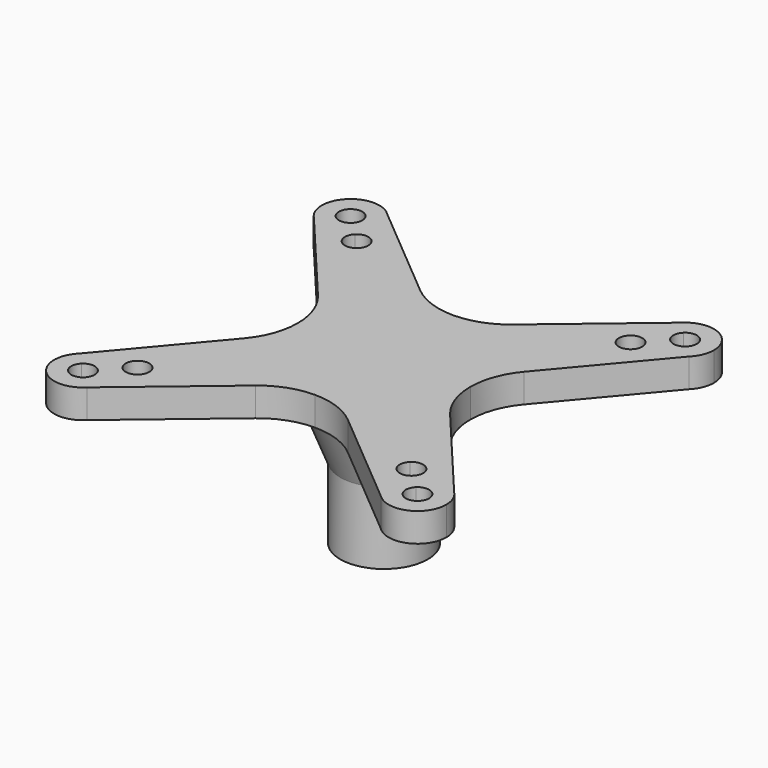
from build123d import *

# Parameters (mm, degrees)
F1_DEPTH = 2.032
F2_DEPTH = 4.572
F4_DEPTH = 5.08


# Not quite as in the source:
# - a fillet or chamfer that OpenCascade refuses, or shapes differently, is made with other operations: its cross-section is extruded or revolved along the edge and cut away or added


with BuildPart() as f1:
    # F0 (on Top) → F1 (new body)
    with BuildSketch(Plane.XY):
        with BuildLine():
            Line((-11.2145823858, 12.3820156815), (-10.3614580543, 13.235140013))
            ThreePointArc((-10.3614580543, 13.235140013), (-13.235140013, 13.235140013), (-13.235140013, 10.3614580543))
            Line((-13.235140013, 10.3614580543), (-12.3820156815, 11.2145823858))
            ThreePointArc((-12.3820156815, 11.2145823858), (-12.3820156815, 12.3820156815), (-11.2145823858, 12.3820156815))
        make_face()
        with BuildLine():
            ThreePointArc((13.8302990336, 11.7982990336), (12.5759117682, 13.6756222437), (10.3614580543, 13.235140013))
            Line((10.3614580543, 13.235140013), (11.2145823858, 12.3820156815))
            ThreePointArc((11.2145823858, 12.3820156815), (12.1142042071, 12.5609615877), (12.6237990336, 11.7982990336))
            ThreePointArc((12.6237990336, 11.7982990336), (12.5609615877, 11.4823938602), (12.3820156815, 11.2145823858))
            Line((12.3820156815, 11.2145823858), (13.235140013, 10.3614580543))
            ThreePointArc((13.235140013, 10.3614580543), (13.6756222437, 11.0206862991), (13.8302990336, 11.7982990336))
        make_face()
        with BuildLine():
            ThreePointArc((13.8302990336, -11.7982990336), (13.6756222437, -11.0206862991), (13.235140013, -10.3614580543))
            Line((13.235140013, -10.3614580543), (12.3820156815, -11.2145823858))
            ThreePointArc((12.3820156815, -11.2145823858), (12.5609615877, -11.4823938602), (12.6237990336, -11.7982990336))
            ThreePointArc((12.6237990336, -11.7982990336), (12.1142042071, -12.5609615877), (11.2145823858, -12.3820156815))
            Line((11.2145823858, -12.3820156815), (10.3614580543, -13.235140013))
            ThreePointArc((10.3614580543, -13.235140013), (12.5759117682, -13.6756222437), (13.8302990336, -11.7982990336))
        make_face()
        with BuildLine():
            Line((-12.3820156815, -11.2145823858), (-13.235140013, -10.3614580543))
            ThreePointArc((-13.235140013, -10.3614580543), (-13.235140013, -13.235140013), (-10.3614580543, -13.235140013))
            Line((-10.3614580543, -13.235140013), (-11.2145823858, -12.3820156815))
            ThreePointArc((-11.2145823858, -12.3820156815), (-12.3820156815, -12.3820156815), (-12.3820156815, -11.2145823858))
        make_face()
        with BuildLine():
            Line((-12.3820156815, 11.2145823858), (-13.235140013, 10.3614580543))
            ThreePointArc((-13.235140013, 10.3614580543), (-11.7982990336, 9.7662990336), (-10.3614580543, 10.3614580543))
            Line((-10.3614580543, 10.3614580543), (-11.2145823858, 11.2145823858))
            ThreePointArc((-11.2145823858, 11.2145823858), (-11.7982990336, 10.9727990336), (-12.3820156815, 11.2145823858))
        make_face()
        with BuildLine():
            ThreePointArc((-9.7662990336, 11.7982990336), (-9.9209758236, 12.5759117682), (-10.3614580543, 13.235140013))
            Line((-10.3614580543, 13.235140013), (-11.2145823858, 12.3820156815))
            ThreePointArc((-11.2145823858, 12.3820156815), (-11.0356364796, 12.1142042071), (-10.9727990336, 11.7982990336))
            ThreePointArc((-10.9727990336, 11.7982990336), (-11.0356364796, 11.4823938602), (-11.2145823858, 11.2145823858))
            Line((-11.2145823858, 11.2145823858), (-10.3614580543, 10.3614580543))
            ThreePointArc((-10.3614580543, 10.3614580543), (-9.9209758236, 11.0206862991), (-9.7662990336, 11.7982990336))
        make_face()
        with BuildLine():
            Line((11.2145823858, 12.3820156815), (10.3614580543, 13.235140013))
            ThreePointArc((10.3614580543, 13.235140013), (9.7662990336, 11.7982990336), (10.3614580543, 10.3614580543))
            Line((10.3614580543, 10.3614580543), (11.2145823858, 11.2145823858))
            ThreePointArc((11.2145823858, 11.2145823858), (10.9727990336, 11.7982990336), (11.2145823858, 12.3820156815))
        make_face()
        with BuildLine():
            Line((11.2145823858, 11.2145823858), (10.3614580543, 10.3614580543))
            ThreePointArc((10.3614580543, 10.3614580543), (11.7982990336, 9.7662990336), (13.235140013, 10.3614580543))
            Line((13.235140013, 10.3614580543), (12.3820156815, 11.2145823858))
            ThreePointArc((12.3820156815, 11.2145823858), (11.7982990336, 10.9727990336), (11.2145823858, 11.2145823858))
        make_face()
        with BuildLine():
            Line((12.3820156815, -11.2145823858), (13.235140013, -10.3614580543))
            ThreePointArc((13.235140013, -10.3614580543), (11.7982990336, -9.7662990336), (10.3614580543, -10.3614580543))
            Line((10.3614580543, -10.3614580543), (11.2145823858, -11.2145823858))
            ThreePointArc((11.2145823858, -11.2145823858), (11.7982990336, -10.9727990336), (12.3820156815, -11.2145823858))
        make_face()
        with BuildLine():
            ThreePointArc((10.3614580543, -10.3614580543), (9.7662990336, -11.7982990336), (10.3614580543, -13.235140013))
            Line((10.3614580543, -13.235140013), (11.2145823858, -12.3820156815))
            ThreePointArc((11.2145823858, -12.3820156815), (10.9727990336, -11.7982990336), (11.2145823858, -11.2145823858))
            Line((11.2145823858, -11.2145823858), (10.3614580543, -10.3614580543))
        make_face()
        with BuildLine():
            Line((-11.2145823858, -12.3820156815), (-10.3614580543, -13.235140013))
            ThreePointArc((-10.3614580543, -13.235140013), (-9.9209758236, -12.5759117682), (-9.7662990336, -11.7982990336))
            ThreePointArc((-9.7662990336, -11.7982990336), (-9.9209758236, -11.0206862991), (-10.3614580543, -10.3614580543))
            Line((-10.3614580543, -10.3614580543), (-11.2145823858, -11.2145823858))
            ThreePointArc((-11.2145823858, -11.2145823858), (-11.0356364796, -11.4823938602), (-10.9727990336, -11.7982990336))
            ThreePointArc((-10.9727990336, -11.7982990336), (-11.0356364796, -12.1142042071), (-11.2145823858, -12.3820156815))
        make_face()
        with BuildLine():
            ThreePointArc((-10.3614580543, -10.3614580543), (-11.7982990336, -9.7662990336), (-13.235140013, -10.3614580543))
            Line((-13.235140013, -10.3614580543), (-12.3820156815, -11.2145823858))
            ThreePointArc((-12.3820156815, -11.2145823858), (-11.7982990336, -10.9727990336), (-11.2145823858, -11.2145823858))
            Line((-11.2145823858, -11.2145823858), (-10.3614580543, -10.3614580543))
        make_face()
        with BuildLine():
            Line((-5.2672343618, 5.2672343618), (-3.2639, 7.2705687236))
            Line((-3.2639, 7.2705687236), (-10.3614580543, 13.235140013))
            ThreePointArc((-10.3614580543, 13.235140013), (-9.9209758236, 12.5759117682), (-9.7662990336, 11.7982990336))
            ThreePointArc((-9.7662990336, 11.7982990336), (-9.9209758236, 11.0206862991), (-10.3614580543, 10.3614580543))
            Line((-10.3614580543, 10.3614580543), (-10.2447147247, 10.2447147247))
            ThreePointArc((-10.2447147247, 10.2447147247), (-9.3450929034, 10.4236606309), (-8.8354980768, 9.6609980768))
            ThreePointArc((-8.8354980768, 9.6609980768), (-8.8983355227, 9.3450929034), (-9.077281429, 9.077281429))
            Line((-9.077281429, 9.077281429), (-5.2672343618, 5.2672343618))
        make_face()
        with BuildLine():
            Line((10.3614580543, 13.235140013), (3.2639, 7.2705687236))
            Line((3.2639, 7.2705687236), (5.2672343618, 5.2672343618))
            Line((5.2672343618, 5.2672343618), (9.077281429, 9.077281429))
            ThreePointArc((9.077281429, 9.077281429), (9.077281429, 10.2447147247), (10.2447147247, 10.2447147247))
            Line((10.2447147247, 10.2447147247), (10.3614580543, 10.3614580543))
            ThreePointArc((10.3614580543, 10.3614580543), (9.7662990336, 11.7982990336), (10.3614580543, 13.235140013))
        make_face()
        with BuildLine():
            Line((9.077281429, 9.077281429), (5.2672343618, 5.2672343618))
            Line((5.2672343618, 5.2672343618), (7.2705687236, 3.2639))
            Line((7.2705687236, 3.2639), (13.235140013, 10.3614580543))
            ThreePointArc((13.235140013, 10.3614580543), (11.7982990336, 9.7662990336), (10.3614580543, 10.3614580543))
            Line((10.3614580543, 10.3614580543), (10.2447147247, 10.2447147247))
            ThreePointArc((10.2447147247, 10.2447147247), (10.4236606309, 9.9769032503), (10.4864980768, 9.6609980768))
            ThreePointArc((10.4864980768, 9.6609980768), (9.9769032503, 8.8983355227), (9.077281429, 9.077281429))
        make_face()
        with BuildLine():
            Line((13.235140013, -10.3614580543), (7.2705687236, -3.2639))
            Line((7.2705687236, -3.2639), (5.2672343618, -5.2672343618))
            Line((5.2672343618, -5.2672343618), (9.077281429, -9.077281429))
            ThreePointArc((9.077281429, -9.077281429), (9.9769032503, -8.8983355227), (10.4864980768, -9.6609980768))
            ThreePointArc((10.4864980768, -9.6609980768), (10.4236606309, -9.9769032503), (10.2447147247, -10.2447147247))
            Line((10.2447147247, -10.2447147247), (10.3614580543, -10.3614580543))
            ThreePointArc((10.3614580543, -10.3614580543), (11.7982990336, -9.7662990336), (13.235140013, -10.3614580543))
        make_face()
        with BuildLine():
            Line((5.2672343618, -5.2672343618), (3.2639, -7.2705687236))
            Line((3.2639, -7.2705687236), (10.3614580543, -13.235140013))
            ThreePointArc((10.3614580543, -13.235140013), (9.7662990336, -11.7982990336), (10.3614580543, -10.3614580543))
            Line((10.3614580543, -10.3614580543), (10.2447147247, -10.2447147247))
            ThreePointArc((10.2447147247, -10.2447147247), (9.077281429, -10.2447147247), (9.077281429, -9.077281429))
            Line((9.077281429, -9.077281429), (5.2672343618, -5.2672343618))
        make_face()
        with BuildLine():
            Line((-3.2639, -7.2705687236), (-5.2672343618, -5.2672343618))
            Line((-5.2672343618, -5.2672343618), (-9.077281429, -9.077281429))
            ThreePointArc((-9.077281429, -9.077281429), (-8.8983355227, -9.3450929034), (-8.8354980768, -9.6609980768))
            ThreePointArc((-8.8354980768, -9.6609980768), (-9.3450929034, -10.4236606309), (-10.2447147247, -10.2447147247))
            Line((-10.2447147247, -10.2447147247), (-10.3614580543, -10.3614580543))
            ThreePointArc((-10.3614580543, -10.3614580543), (-9.9209758236, -11.0206862991), (-9.7662990336, -11.7982990336))
            ThreePointArc((-9.7662990336, -11.7982990336), (-9.9209758236, -12.5759117682), (-10.3614580543, -13.235140013))
            Line((-10.3614580543, -13.235140013), (-3.2639, -7.2705687236))
        make_face()
        with BuildLine():
            Line((-7.2705687236, 3.2639), (-5.2672343618, 5.2672343618))
            Line((-5.2672343618, 5.2672343618), (-9.077281429, 9.077281429))
            ThreePointArc((-9.077281429, 9.077281429), (-10.2447147247, 9.077281429), (-10.2447147247, 10.2447147247))
            Line((-10.2447147247, 10.2447147247), (-10.3614580543, 10.3614580543))
            ThreePointArc((-10.3614580543, 10.3614580543), (-11.7982990336, 9.7662990336), (-13.235140013, 10.3614580543))
            Line((-13.235140013, 10.3614580543), (-7.2705687236, 3.2639))
        make_face()
        with BuildLine():
            Line((-5.2672343618, -5.2672343618), (-7.2705687236, -3.2639))
            Line((-7.2705687236, -3.2639), (-13.235140013, -10.3614580543))
            ThreePointArc((-13.235140013, -10.3614580543), (-11.7982990336, -9.7662990336), (-10.3614580543, -10.3614580543))
            Line((-10.3614580543, -10.3614580543), (-10.2447147247, -10.2447147247))
            ThreePointArc((-10.2447147247, -10.2447147247), (-10.2447147247, -9.077281429), (-9.077281429, -9.077281429))
            Line((-9.077281429, -9.077281429), (-5.2672343618, -5.2672343618))
        make_face()
        with BuildLine():
            ThreePointArc((3.2639, 7.2705687236), (1.7365663126, 6.3893354587), (0, 6.0833))
            Line((0, 6.0833), (0, 4.8641))
            ThreePointArc((0, 4.8641), (3.4394380944, 3.4394380944), (4.8641, 0))
            Line((4.8641, 0), (6.0833, 0))
            ThreePointArc((6.0833, 0), (6.3893354587, 1.7365663126), (7.2705687236, 3.2639))
            Line((7.2705687236, 3.2639), (5.2672343618, 5.2672343618))
            Line((5.2672343618, 5.2672343618), (3.2639, 7.2705687236))
        make_face()
        with BuildLine():
            Line((0, 4.8641), (0, 6.0833))
            ThreePointArc((0, 6.0833), (-1.7365663126, 6.3893354587), (-3.2639, 7.2705687236))
            Line((-3.2639, 7.2705687236), (-5.2672343618, 5.2672343618))
            Line((-5.2672343618, 5.2672343618), (-7.2705687236, 3.2639))
            ThreePointArc((-7.2705687236, 3.2639), (-6.3893354587, 1.7365663126), (-6.0833, 0))
            Line((-6.0833, 0), (-4.8641, 0))
            ThreePointArc((-4.8641, 0), (-3.4394380944, 3.4394380944), (0, 4.8641))
        make_face()
        with BuildLine():
            Line((0, -4.8641), (0, 0))
            Line((0, 0), (-4.8641, 0))
            ThreePointArc((-4.8641, 0), (-3.4394380944, -3.4394380944), (0, -4.8641))
        make_face()
        with BuildLine():
            Line((4.8641, 0), (0, 0))
            Line((0, 0), (0, -4.8641))
            ThreePointArc((0, -4.8641), (3.4394380944, -3.4394380944), (4.8641, 0))
        make_face()
        with BuildLine():
            Line((5.2672343618, -5.2672343618), (7.2705687236, -3.2639))
            ThreePointArc((7.2705687236, -3.2639), (6.3893354587, -1.7365663126), (6.0833, 0))
            Line((6.0833, 0), (4.8641, 0))
            ThreePointArc((4.8641, 0), (3.4394380944, -3.4394380944), (0, -4.8641))
            Line((0, -4.8641), (0, -6.0833))
            ThreePointArc((0, -6.0833), (1.7365663126, -6.3893354587), (3.2639, -7.2705687236))
            Line((3.2639, -7.2705687236), (5.2672343618, -5.2672343618))
        make_face()
        with BuildLine():
            ThreePointArc((-6.0833, 0), (-6.3893354587, -1.7365663126), (-7.2705687236, -3.2639))
            Line((-7.2705687236, -3.2639), (-5.2672343618, -5.2672343618))
            Line((-5.2672343618, -5.2672343618), (-3.2639, -7.2705687236))
            ThreePointArc((-3.2639, -7.2705687236), (-1.7365663126, -6.3893354587), (0, -6.0833))
            Line((0, -6.0833), (0, -4.8641))
            ThreePointArc((0, -4.8641), (-3.4394380944, -3.4394380944), (-4.8641, 0))
            Line((-4.8641, 0), (-6.0833, 0))
        make_face()
        with BuildLine():
            Line((0, 0), (0, 4.8641))
            ThreePointArc((0, 4.8641), (-3.4394380944, 3.4394380944), (-4.8641, 0))
            Line((-4.8641, 0), (0, 0))
        make_face()
        with BuildLine():
            ThreePointArc((4.8641, 0), (3.4394380944, 3.4394380944), (0, 4.8641))
            Line((0, 4.8641), (0, 0))
            Line((0, 0), (4.8641, 0))
        make_face()
    extrude(amount=F1_DEPTH)

    # F0 (on Top) → F2 (join)
    with BuildSketch(Plane.XY):
        with BuildLine():
            Line((0, 0), (0, 4.8641))
            ThreePointArc((0, 4.8641), (-3.4394380944, 3.4394380944), (-4.8641, 0))
            Line((-4.8641, 0), (0, 0))
        make_face()
        with BuildLine():
            Line((4.8641, 0), (0, 0))
            Line((0, 0), (0, -4.8641))
            ThreePointArc((0, -4.8641), (3.4394380944, -3.4394380944), (4.8641, 0))
        make_face()
        with BuildLine():
            ThreePointArc((4.8641, 0), (3.4394380944, 3.4394380944), (0, 4.8641))
            Line((0, 4.8641), (0, 0))
            Line((0, 0), (4.8641, 0))
        make_face()
        with BuildLine():
            Line((0, -4.8641), (0, 0))
            Line((0, 0), (-4.8641, 0))
            ThreePointArc((-4.8641, 0), (-3.4394380944, -3.4394380944), (0, -4.8641))
        make_face()
    extrude(amount=-F2_DEPTH)

    # F3: chamfer of 4.572 x 1.778 on 1 edges, made by hand


with BuildPart() as f3_tool2:
    # F3_s3 → F3_t4 (revolve)
    with BuildSketch(Plane.XZ):
        Polygon((-4.8641, 0), (-3.0861, -4.572), (-4.8641, -4.572), align=None)
    revolve(axis=Axis((0, 0, -4.572), (0, 0, 1)))

    split(bisect_by=Plane.XY, keep=Keep.BOTTOM)


with BuildPart() as f1_1:
    add(f1.part)

    # F3_t1: cut F3_tool2
    add(f3_tool2.part, mode=Mode.SUBTRACT)

    # F4 (add): a face of the model
    f4_faces = [f1_1.faces().sort_by_distance(p)[0] for p in [
        (0, 0, -4.572),
    ]]
    extrude(f4_faces, amount=F4_DEPTH)


solid = f1_1.part
